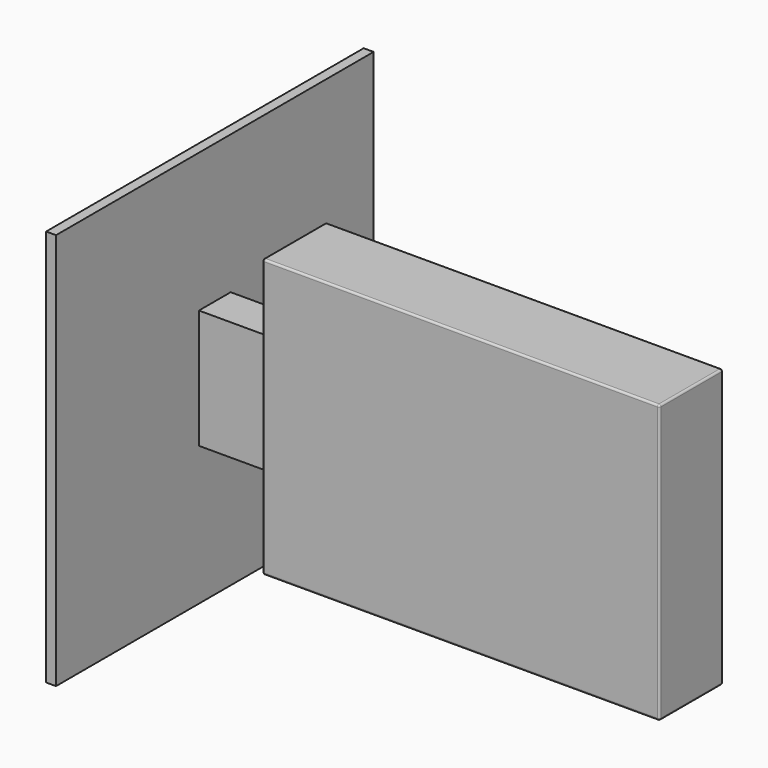
from build123d import *

# Parameters (mm, degrees)
F0_W     = 1000
F0_H     = 1000
F1_DEPTH = 25
F2_W     = 100
F2_H     = 300
F3_DEPTH = 200
F4_W     = 200
F4_H     = 700
F4_W_2   = 100
F4_H_2   = 300
F5_DEPTH = 1000
F6_R     = 5


# Not quite as in the source:
# - two fillets or chamfers of one size are made in one step


with BuildPart() as f1:
    # F0 (on Right) → F1 (new body)
    with BuildSketch(Plane.YZ):
        with Locations((334.907528758, 427.1594434977)):
            Rectangle(F0_W, F0_H)
    extrude(amount=F1_DEPTH)

    # F2 (on face) → F3 (join)
    with BuildSketch(Plane.YZ.offset(25)):
        with Locations((334.907528758, 427.1594434977)):
            Rectangle(F2_W, F2_H)
    extrude(amount=F3_DEPTH)

    # F4 (on face) → F5 (join)
    with BuildSketch(Plane.YZ.offset(225)):
        with Locations((334.907528758, 427.1594434977)):
            Rectangle(F4_W, F4_H)
        with Locations((334.907528758, 427.1594434977)):
            Rectangle(F4_W_2, F4_H_2, mode=Mode.SUBTRACT)
        with Locations((334.907528758, 427.1594434977)):
            Rectangle(F4_W_2, F4_H_2)
    extrude(amount=F5_DEPTH)

    # F6
    f6_edges = [f1.edges().sort_by_distance(p)[0] for p in [
        (225, 234.907529, 427.159443),
        (225, 284.907529, 427.159443),
        (725, 234.907529, 777.159443),
        (1225, 234.907529, 427.159443),
        (1225, 334.907529, 777.159443),
        (725, 234.907529, 77.159443),
        (225, 334.907529, 77.159443),
        (1225, 334.907529, 77.159443),
        (225, 334.907529, 777.159443),
        (725, 434.907529, 77.159443),
        (725, 434.907529, 777.159443),
        (225, 434.907529, 427.159443),
        (1225, 434.907529, 427.159443),
    ]]
    fillet(f6_edges, radius=F6_R)


solid = f1.part
